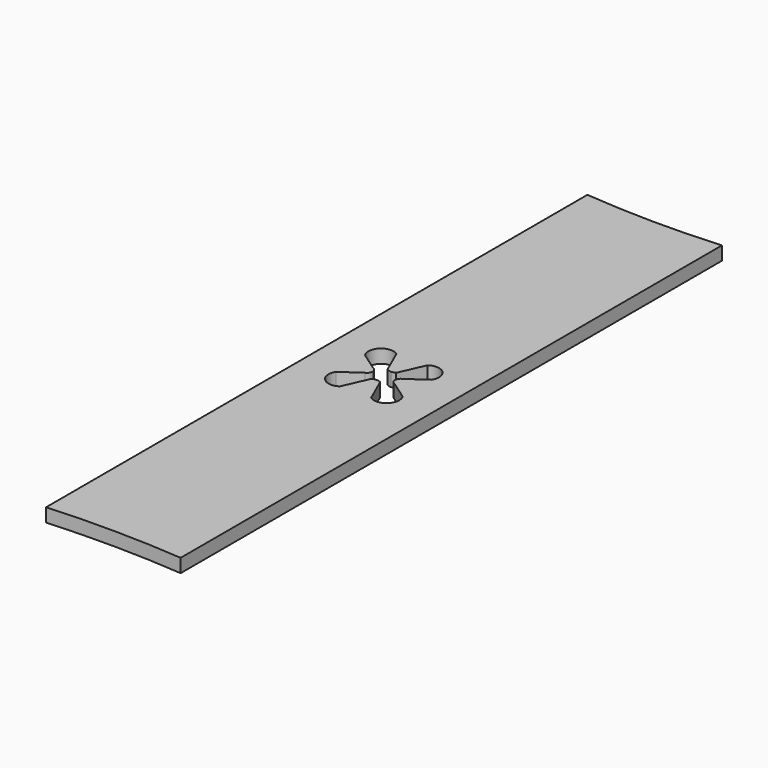
from build123d import *

# Parameters (mm, degrees)
F1_DEPTH = 25.4
F3_DEPTH = 25.4
F4_DEPTH = 25.4


# Not quite as in the source:
# - a feature names something its author has since deleted; it is built from what else it names


with BuildPart() as f1:
    # F0 (on Top) → F1 (new body)
    with BuildSketch(Plane.XY):
        with BuildLine():
            ThreePointArc((128.3595710993, 553.8759422302), (1.1825358552, 549.8230168828), (-125.9080190212, 556.0210293531))
            Line((-125.9080190212, 556.0210293531), (-125.9080190212, -713.9789706469))
            ThreePointArc((-125.9080190212, -713.9789706469), (1.2643600135, -710.4779684085), (128.3595710993, -716.1240577698))
            Line((128.3595710993, -716.1240577698), (128.3595710993, 553.8759422302))
        make_face()
    extrude(amount=F1_DEPTH)

    # F2 (on face) → F3 (cut, through all)
    with BuildSketch(Plane.XY.offset(25.4)):
        with BuildLine():
            Line((21.1381499791, -78.9789706469), (0, -78.9789706469))
            Line((0, -78.9789706469), (0, -95.7576301918))
            ThreePointArc((0, -95.7576301918), (4.2283594629, -96.2864641581), (8.1962319091, -97.8403873742))
            Line((8.1962319091, -97.8403873742), (29.1618719602, -145.247048063))
            ThreePointArc((29.1618719602, -145.247048063), (59.1063769686, -142.7132397651), (62.4383196322, -112.8470092903))
            Line((62.4383196322, -112.8470092903), (27.7889794812, -88.7078500401))
            ThreePointArc((27.7889794812, -88.7078500401), (22.9597605864, -84.8714367544), (21.1381499791, -78.9789706469))
        make_face()
        with BuildLine():
            Line((0, -78.9789706469), (-21.1381499791, -78.9789706469))
            ThreePointArc((-21.1381499791, -78.9789706469), (-22.9597605864, -84.8714367544), (-27.7889794812, -88.7078500401))
            Line((-27.7889794812, -88.7078500401), (-62.4383196322, -112.8470092903))
            ThreePointArc((-62.4383196322, -112.8470092903), (-59.1063769686, -142.7132397651), (-29.1618719602, -145.247048063))
            Line((-29.1618719602, -145.247048063), (-8.3430390852, -97.9210786899))
            ThreePointArc((-8.3430390852, -97.9210786899), (-4.3094898358, -96.30729114), (0, -95.7576301918))
            Line((0, -95.7576301918), (0, -78.9789706469))
        make_face()
    extrude(amount=-F3_DEPTH, mode=Mode.SUBTRACT)

    # F2 (on face) → F4 (cut, through all)
    with BuildSketch(Plane.XY.offset(25.4)):
        with BuildLine():
            ThreePointArc((-27.7889794812, -69.2500912536), (-22.9597605864, -73.0865045393), (-21.1381499791, -78.9789706469))
            Line((-21.1381499791, -78.9789706469), (0, -78.9789706469))
            Line((0, -78.9789706469), (0, -62.2003111019))
            ThreePointArc((0, -62.2003111019), (-4.3094898358, -61.6506501538), (-8.3430390852, -60.0368626038))
            Line((-8.3430390852, -60.0368626038), (-29.1618719602, -12.7108932307))
            ThreePointArc((-29.1618719602, -12.7108932307), (-59.1063769686, -15.2447015287), (-62.4383196322, -45.1109320034))
            Line((-62.4383196322, -45.1109320034), (-27.7889794812, -69.2500912536))
        make_face()
        with BuildLine():
            Line((0, -62.2003111019), (0, -78.9789706469))
            Line((0, -78.9789706469), (21.1381499791, -78.9789706469))
            ThreePointArc((21.1381499791, -78.9789706469), (22.9597605864, -73.0865045393), (27.7889794812, -69.2500912536))
            Line((27.7889794812, -69.2500912536), (62.4383196322, -45.1109320034))
            ThreePointArc((62.4383196322, -45.1109320034), (59.1063769686, -15.2447015287), (29.1618719602, -12.7108932307))
            Line((29.1618719602, -12.7108932307), (8.1962319091, -60.1175539196))
            ThreePointArc((8.1962319091, -60.1175539196), (4.2283594629, -61.6714771356), (0, -62.2003111019))
        make_face()
    extrude(amount=-F4_DEPTH, mode=Mode.SUBTRACT)


solid = f1.part
